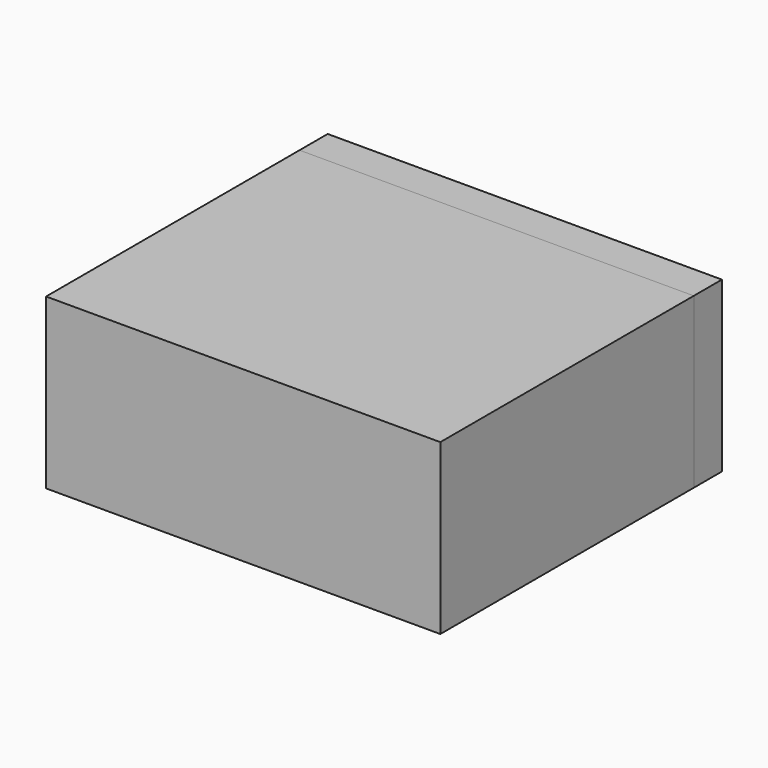
from build123d import *

# Parameters (mm, degrees)
F0_W     = 177.8
F0_H     = 142.875
F1_DEPTH = 76.2
F2_DEPTH = 15.875


# Not quite as in the source:
# - a length typed as a fraction of an inch, garbled in the dataset ("3 / 203.2 mm" for 3/8 in), is restored


with BuildPart() as f1:
    # F0 (on Top) → F1 (new body)
    with BuildSketch(Plane.XY):
        with Locations((-6.3983104533, -14.8231089294)):
            Rectangle(F0_W, F0_H)
    extrude(amount=F1_DEPTH)


with BuildPart() as f2:
    # F2 (new): a face of the model
    f2_faces = [f1.part.faces().sort_by_distance(p)[0] for p in [
        (-6.3983104533, 56.6143910706, 38.1),
    ]]
    extrude(f2_faces, amount=F2_DEPTH)


solid = Compound([f1.part, f2.part])
